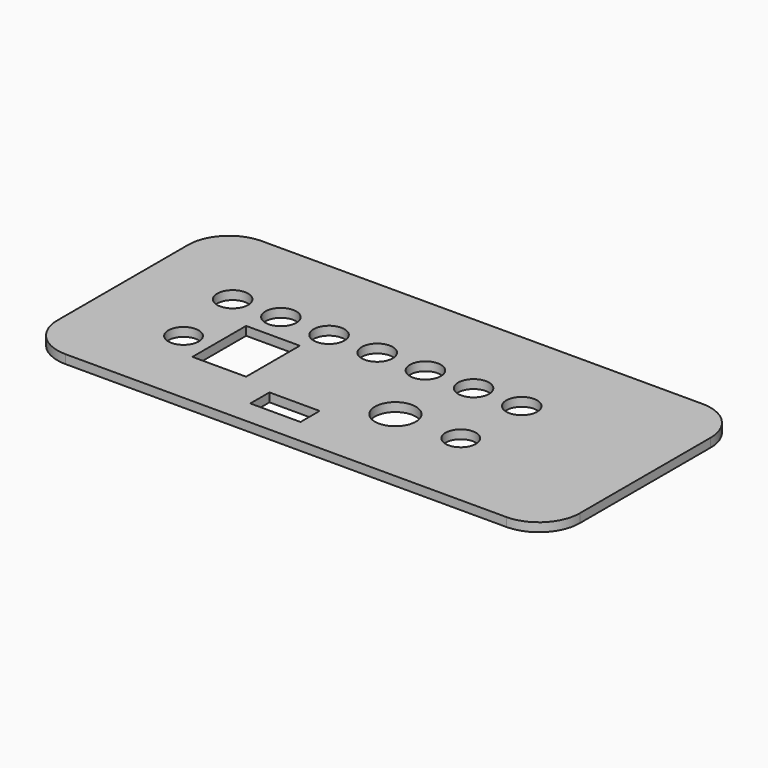
from build123d import *

# Parameters (mm, degrees)
F0_W     = 8.6
F0_H     = 4.1
F0_W_2   = 9.2
F0_H_2   = 11.5
F1_DEPTH = 1.5
F2_D     = 5.2
F2_DEPTH = 2
F2_TIP   = 1.5622376095
F3_D     = 7
F3_DEPTH = 2
F3_TIP   = 2.1030121666
F4_D     = 5.3
F4_DEPTH = 2
F4_TIP   = 1.5922806404


# Not quite as in the source:
# - a feature names something its author has since deleted; it is built from what else it names


with BuildPart() as f1:
    # F0 (on Top) → F1 (new body)
    with BuildSketch(Plane.XY):
        with BuildLine():
            Line((-37.75, -21), (37.75, -21))
            ThreePointArc((37.75, -21), (42.6997474683, -18.9497474683), (44.75, -14))
            Line((44.75, -14), (44.75, 14))
            ThreePointArc((44.75, 14), (42.6997474683, 18.9497474683), (37.75, 21))
            Line((37.75, 21), (-37.75, 21))
            ThreePointArc((-37.75, 21), (-42.6997474683, 18.9497474683), (-44.75, 14))
            Line((-44.75, 14), (-44.75, -14))
            ThreePointArc((-44.75, -14), (-42.6997474683, -18.9497474683), (-37.75, -21))
        make_face()
        with Locations((-5.25, -14.65)):
            Rectangle(F0_W, F0_H, mode=Mode.SUBTRACT)
        with Locations((-19.43, -5.25)):
            Rectangle(F0_W_2, F0_H_2, mode=Mode.SUBTRACT)
    extrude(amount=F1_DEPTH)

    # F2
    with Locations(Plane(origin=(0, 0, 0), x_dir=(1, 0, 0), z_dir=(0, 0, -1))):
        with Locations((18.75, 7), (-28.75, 7)):
            Hole(F2_D / 2, depth=F2_DEPTH)
            with Locations((0, 0, -(F2_DEPTH + F2_TIP / 2))):  # 118° drill point
                Cone(0, F2_D / 2, F2_TIP, mode=Mode.SUBTRACT)

    # F3
    with Locations(Plane(origin=(0, 0, 0), x_dir=(1, 0, 0), z_dir=(0, 0, -1))):
        with Locations((7.55, 7)):
            Hole(F3_D / 2, depth=F3_DEPTH)
            with Locations((0, 0, -(F3_DEPTH + F3_TIP / 2))):  # 118° drill point
                Cone(0, F3_D / 2, F3_TIP, mode=Mode.SUBTRACT)

    # F4
    with Locations(Plane(origin=(0, 0, 0), x_dir=(1, 0, 0), z_dir=(0, 0, -1))):
        with Locations((-30.2482247353, -5.4), (-21.9932247353, -5.4), (-13.7382247353, -5.4), (-5.4832247353, -5.4), (2.7717752647, -5.4), (11.0267752647, -5.4), (19.2817752647, -5.4)):
            Hole(F4_D / 2, depth=F4_DEPTH)
            with Locations((0, 0, -(F4_DEPTH + F4_TIP / 2))):  # 118° drill point
                Cone(0, F4_D / 2, F4_TIP, mode=Mode.SUBTRACT)


solid = f1.part
